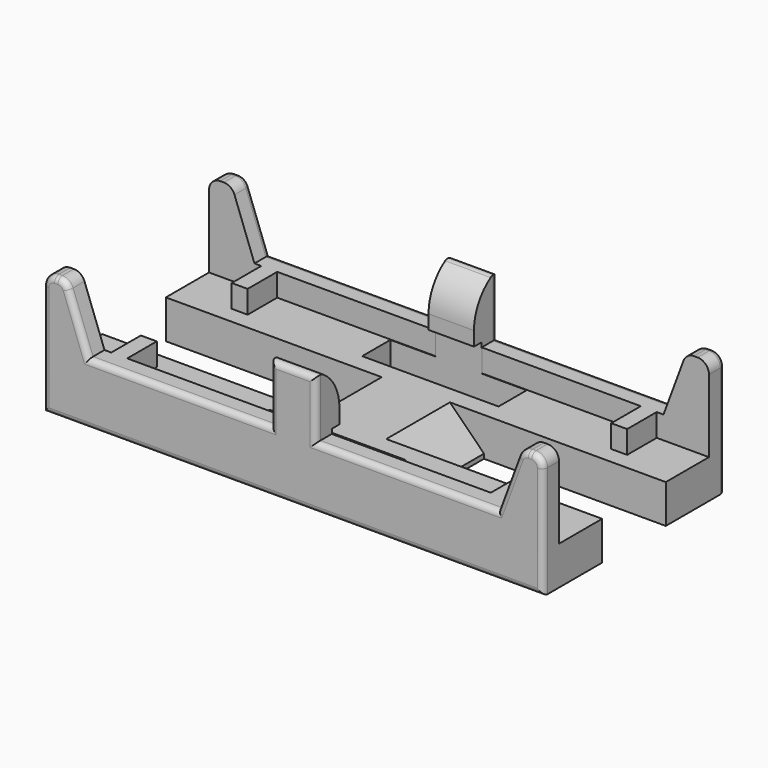
from build123d import *

# Parameters (mm, degrees)
F0_W         = 55.88
F0_H         = 25.4
F1_DEPTH     = 13.716
F2_W         = 20.32
F2_H         = 8.89
F3_DEPTH     = 13.717
F4_W         = 20.32
F4_H         = 8.89
F5_DEPTH     = 13.717
F6_W         = 15.24
F6_H         = 3.937
F7_DEPTH     = 7.366
F8_W         = 15.24
F8_H         = 3.937
F9_DEPTH     = 7.366
F10_W        = 55.88
F10_H        = 18.796
F11_DEPTH    = 9.398
F12_W        = 20.32
F12_H        = 6.858
F13_DEPTH    = 25.401
F14_W        = 20.32
F14_H        = 6.858
F15_DEPTH    = 25.401
F17_DEPTH    = 25.401
F19_DEPTH    = 25.401
F20_R        = 1.27
F21_W        = 38.1
F21_H        = 20.955
F22_DEPTH    = 9.398
F23_W        = 38.1
F23_H        = 20.955
F24_DEPTH    = 9.398
F25_T1_DEPTH = 28.8734423739
F26_W        = 1.778
F26_H        = 20.955
F27_DEPTH    = 2.54
F28_W        = 1.778
F28_H        = 20.955
F29_DEPTH    = 2.54
F30_W        = 55.88
F30_H        = 12.7
F31_DEPTH    = 2.54
F32_SIZE     = 3.81
F33_R        = 0.635


# Not quite as in the source:
# - a fillet or chamfer that OpenCascade refuses, or shapes differently, is made with other operations: its cross-section is extruded or revolved along the edge and cut away or added


with BuildPart() as f1:
    # F0 (on Top) → F1 (new body)
    with BuildSketch(Plane.XY):
        Rectangle(F0_W, F0_H)
    extrude(amount=F1_DEPTH)

    # F2 (on face) → F3 (cut, through all)
    with BuildSketch(Plane(origin=(0, 0, 0), x_dir=(1, 0, 0), z_dir=(0, 0, -1))):
        with Locations((17.78, 0)):
            Rectangle(F2_W, F2_H)
    extrude(amount=-F3_DEPTH, mode=Mode.SUBTRACT)

    # F4 (on face) → F5 (cut, through all)
    with BuildSketch(Plane(origin=(0, 0, 0), x_dir=(1, 0, 0), z_dir=(0, 0, -1))):
        with Locations((-17.78, 0)):
            Rectangle(F4_W, F4_H)
    extrude(amount=-F5_DEPTH, mode=Mode.SUBTRACT)

    # F6 (on face) → F7 (cut)
    with BuildSketch(Plane(origin=(0, 0, 0), x_dir=(1, 0, 0), z_dir=(0, 0, -1))):
        with Locations((0, 8.4455)):
            Rectangle(F6_W, F6_H)
    extrude(amount=-F7_DEPTH, mode=Mode.SUBTRACT)

    # F8 (on face) → F9 (cut)
    with BuildSketch(Plane(origin=(0, 0, 0), x_dir=(1, 0, 0), z_dir=(0, 0, -1))):
        with Locations((0, -8.4455)):
            Rectangle(F8_W, F8_H)
    extrude(amount=-F9_DEPTH, mode=Mode.SUBTRACT)

    # F10 (on face) → F11 (cut)
    with BuildSketch(Plane.XY.offset(13.716)):
        Rectangle(F10_W, F10_H)
    extrude(amount=-F11_DEPTH, mode=Mode.SUBTRACT)

    # F12 (on face) → F13 (cut, through all)
    with BuildSketch(Plane.XZ.offset(12.7)):
        with Locations((-12.7, 10.287)):
            Rectangle(F12_W, F12_H)
    extrude(amount=-F13_DEPTH, mode=Mode.SUBTRACT)

    # F14 (on face) → F15 (cut, through all)
    with BuildSketch(Plane.XZ.offset(12.7)):
        with Locations((12.7, 10.287)):
            Rectangle(F14_W, F14_H)
    extrude(amount=-F15_DEPTH, mode=Mode.SUBTRACT)

    # F16 (on face) → F17 (cut, through all)
    with BuildSketch(Plane.XZ.offset(12.7)):
        Polygon((-25.4, 13.716), (-22.86, 6.858), (-22.86, 13.716), align=None)
    extrude(amount=-F17_DEPTH, mode=Mode.SUBTRACT)

    # F18 (on face) → F19 (cut, through all)
    with BuildSketch(Plane.XZ.offset(12.7)):
        Polygon((22.86, 13.716), (22.86, 6.858), (25.4, 13.716), align=None)
    extrude(amount=-F19_DEPTH, mode=Mode.SUBTRACT)

    # F20
    f20_edges = [f1.edges().sort_by_distance(p)[0] for p in [
        (-25.4, 11.049, 13.716),
        (-25.4, -11.049, 13.716),
        (25.4, 11.049, 13.716),
        (25.4, -11.049, 13.716),
        (-27.94, 11.049, 13.716),
        (-27.94, -11.049, 13.716),
        (27.94, -11.049, 13.716),
        (27.94, 11.049, 13.716),
    ]]
    fillet(f20_edges, radius=F20_R)

    # F21 (on face) → F22 (cut)
    with BuildSketch(Plane.XY.offset(13.716)):
        with Locations((-21.6148423028, 0)):
            Rectangle(F21_W, F21_H)
    extrude(amount=-F22_DEPTH, mode=Mode.SUBTRACT)

    # F23 (on face) → F24 (cut)
    with BuildSketch(Plane.XY.offset(13.716)):
        with Locations((21.6445253996, 0)):
            Rectangle(F23_W, F23_H)
    extrude(amount=-F24_DEPTH, mode=Mode.SUBTRACT)

    # F25: fillet of radius 5.08 on 2 edges, made by hand

    # F25_s2 → F25_t1 (cut)
    with BuildSketch(Plane.YZ.offset(-14.4367211869)):
        with BuildLine():
            ThreePointArc((9.398, 8.9573115252), (10.3043541118, 11.853357105), (12.7, 13.716))
            Line((12.7, 13.716), (9.398, 13.716))
            Line((9.398, 13.716), (9.398, 8.9573115252))
        make_face()
        with BuildLine():
            ThreePointArc((-12.7, 13.716), (-10.3043541118, 11.853357105), (-9.398, 8.9573115252))
            Line((-9.398, 8.9573115252), (-9.398, 13.716))
            Line((-9.398, 13.716), (-12.7, 13.716))
        make_face()
    extrude(amount=F25_T1_DEPTH, mode=Mode.SUBTRACT)

    # F26 (on face) → F27 (join)
    with BuildSketch(Plane.XY.offset(4.318)):
        with Locations((21.209, 0)):
            Rectangle(F26_W, F26_H)
    extrude(amount=F27_DEPTH)

    # F28 (on face) → F29 (join)
    with BuildSketch(Plane.XY.offset(4.318)):
        with Locations((-21.209, 0)):
            Rectangle(F28_W, F28_H)
    extrude(amount=F29_DEPTH)

    # F30 (on face) → F31 (cut)
    with BuildSketch(Plane.XY.offset(6.858)):
        with Locations((-0.1600864343, 0)):
            Rectangle(F30_W, F30_H)
    extrude(amount=-F31_DEPTH, mode=Mode.SUBTRACT)

    # F32
    f32_edges = [f1.edges().sort_by_distance(p)[0] for p in [
        (7.62, 0, 4.318),
        (-7.62, 0, 4.318),
    ]]
    chamfer(f32_edges, length=F32_SIZE)

    # F33
    f33_edges = [f1.edges().sort_by_distance(p)[0] for p in [
        (27.94, -12.7, 6.223),
        (27.568026, -12.7, 13.344026),
        (0, -12.7, 0),
        (26.476968, -12.7, 13.716),
        (-27.94, -12.7, 6.223),
        (25.558431, -12.7, 13.488373),
        (-27.568026, -12.7, 13.344026),
        (23.976498, -12.7, 9.872545),
        (-26.476968, -12.7, 13.716),
        (12.7, -12.7, 6.858),
        (-25.558431, -12.7, 13.488373),
        (2.54, -12.7, 10.287),
        (-23.976498, -12.7, 9.872545),
        (0, -12.7, 13.716),
        (-12.7, -12.7, 6.858),
        (-2.54, -12.7, 10.287),
        (-27.94, 12.7, 6.223),
        (-27.568026, 12.7, 13.344026),
        (0, 12.7, 0),
        (-26.476968, 12.7, 13.716),
        (27.94, 12.7, 6.223),
        (-25.558431, 12.7, 13.488373),
        (27.568026, 12.7, 13.344026),
        (-23.976498, 12.7, 9.872545),
        (26.476968, 12.7, 13.716),
        (-12.7, 12.7, 6.858),
        (25.558431, 12.7, 13.488373),
        (-2.54, 12.7, 10.287),
        (23.976498, 12.7, 9.872545),
        (0, 12.7, 13.716),
        (12.7, 12.7, 6.858),
        (2.54, 12.7, 10.287),
    ]]
    fillet(f33_edges, radius=F33_R)


solid = f1.part
